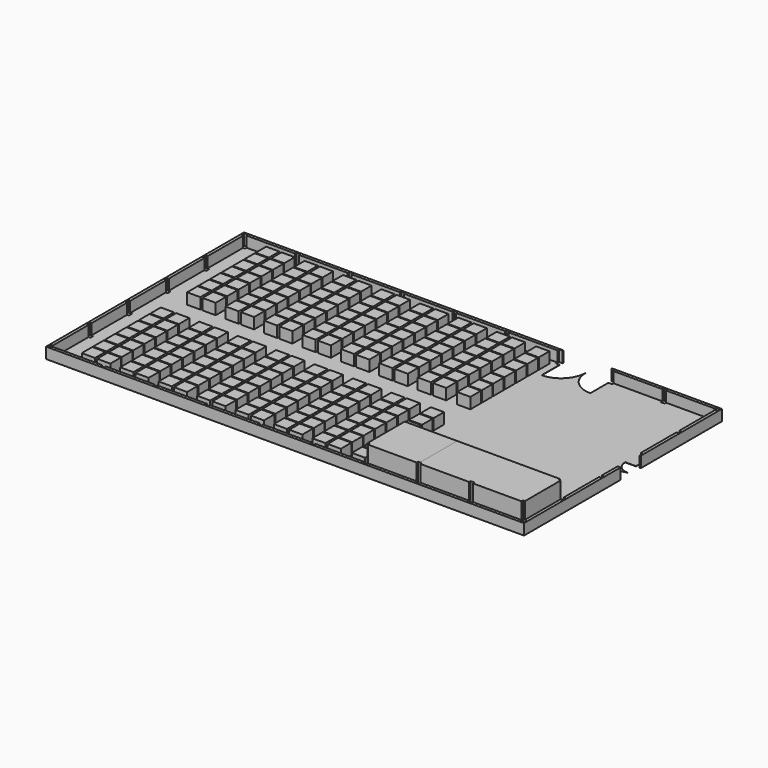
from build123d import *

# Parameters (mm, degrees)
F1_DEPTH = 25
F2_DEPTH = 2500
F3_DEPTH = 2500
F4_DEPTH = 1000
F5_W     = 1200
F5_H     = 1200
F6_DEPTH = 1000


# Not quite as in the source:
# - a feature names something its author has since deleted; it is built from what else it names


with BuildPart() as f1:
    # F0 (on Top) → F1 (new body)
    with BuildSketch(Plane.XY):
        Polygon((28666.6668, 170), (28666.6668, 4400), (28666.6668, 10000), (0, 10000), (0, 8970), (170, 8970), (170, 8630), (0, 8630), (0, 4570), (170, 4570), (170, 4230), (0, 4230), (0, 170), (170, 170), (170, 0), (4607.7778, 0), (4607.7778, 170), (4947.7778, 170), (4947.7778, 0), (9385.5556, 0), (9385.5556, 170), (9725.5556, 170), (9725.5556, 0), (14163.3334, 0), (14163.3334, 170), (14503.3334, 170), (14503.3334, 0), (18941.1112, 0), (18941.1112, 170), (19281.1112, 170), (19281.1112, 0), (23718.889, 0), (23718.889, 170), (24058.889, 170), (24058.889, 0), (28496.6668, 0), (28496.6668, 170), align=None)
        with BuildLine():
            ThreePointArc((33274.4446, 19781.1111), (31705.4532121104, 20431.0086121104), (31055.5557, 22000))
            ThreePointArc((31055.5557, 22000), (30405.6581878896, 20431.0086121104), (28836.6668, 19781.1111))
            Line((28836.6668, 19781.1111), (28836.6668, 21830))
            Line((28836.6668, 21830), (28496.6668, 21830))
            Line((28496.6668, 21830), (28496.6668, 22000))
            Line((28496.6668, 22000), (24058.889, 22000))
            Line((24058.889, 22000), (24058.889, 21830))
            Line((24058.889, 21830), (23718.889, 21830))
            Line((23718.889, 21830), (23718.889, 22000))
            Line((23718.889, 22000), (19281.1112, 22000))
            Line((19281.1112, 22000), (19281.1112, 21830))
            Line((19281.1112, 21830), (18941.1112, 21830))
            Line((18941.1112, 21830), (18941.1112, 22000))
            Line((18941.1112, 22000), (14503.3334, 22000))
            Line((14503.3334, 22000), (14503.3334, 21830))
            Line((14503.3334, 21830), (14163.3334, 21830))
            Line((14163.3334, 21830), (14163.3334, 22000))
            Line((14163.3334, 22000), (9725.5556, 22000))
            Line((9725.5556, 22000), (9725.5556, 21830))
            Line((9725.5556, 21830), (9385.5556, 21830))
            Line((9385.5556, 21830), (9385.5556, 22000))
            Line((9385.5556, 22000), (4947.7778, 22000))
            Line((4947.7778, 22000), (4947.7778, 21830))
            Line((4947.7778, 21830), (4607.7778, 21830))
            Line((4607.7778, 21830), (4607.7778, 22000))
            Line((4607.7778, 22000), (170, 22000))
            Line((170, 22000), (170, 21830))
            Line((170, 21830), (0, 21830))
            Line((0, 21830), (0, 17770))
            Line((0, 17770), (170, 17770))
            Line((170, 17770), (170, 17430))
            Line((170, 17430), (0, 17430))
            Line((0, 17430), (0, 13370))
            Line((0, 13370), (170, 13370))
            Line((170, 13370), (170, 13030))
            Line((170, 13030), (0, 13030))
            Line((0, 13030), (0, 12000))
            Line((0, 12000), (0, 10000))
            Line((0, 10000), (28666.6668, 10000))
            Line((28666.6668, 10000), (28666.6668, 4400))
            Line((28666.6668, 4400), (33444.4446, 4400))
            Line((33444.4446, 4400), (42830, 4400))
            Line((42830, 4400), (42830, 4570))
            Line((42830, 4570), (43000, 4570))
            Line((43000, 4570), (43000, 8630))
            Line((43000, 8630), (42830, 8630))
            Line((42830, 8630), (42830, 8970))
            Line((42830, 8970), (43000, 8970))
            Line((43000, 8970), (43000, 10730))
            Line((43000, 10730), (41850, 10730))
            ThreePointArc((41850, 10730), (42186.8272016355, 11543.1727983645), (43000, 11880))
            ThreePointArc((43000, 11880), (42186.8272016355, 12216.8272016355), (41850, 13030))
            Line((41850, 13030), (42830, 13030))
            Line((42830, 13030), (42830, 13370))
            Line((42830, 13370), (43000, 13370))
            Line((43000, 13370), (43000, 17430))
            Line((43000, 17430), (42830, 17430))
            Line((42830, 17430), (42830, 17770))
            Line((42830, 17770), (43000, 17770))
            Line((43000, 17770), (43000, 21830))
            Line((43000, 21830), (42830.0002, 21830))
            Line((42830.0002, 21830), (42830.0002, 22000))
            Line((42830.0002, 22000), (38392.2224, 22000))
            Line((38392.2224, 22000), (38392.2224, 21830))
            Line((38392.2224, 21830), (38052.2224, 21830))
            Line((38052.2224, 21830), (38052.2224, 22000))
            Line((38052.2224, 22000), (33614.4446, 22000))
            Line((33614.4446, 22000), (33614.4446, 21830))
            Line((33614.4446, 21830), (33274.4446, 21830))
            Line((33274.4446, 21830), (33274.4446, 19781.1111))
        make_face()
    extrude(amount=F1_DEPTH)

    # F0 (on Top) → F4 (join)
    with BuildSketch(Plane.XY):
        Polygon((24058.889, 22000), (28496.6668, 22000), (28496.6668, 22170), (28836.6668, 22170), (28836.6668, 22270), (-270, 22270), (-270, -270), (43270.0002, -270), (43270.0002, 10730), (43000, 10730), (43000, 8970), (43170, 8970), (43170, 8630), (43000, 8630), (43000, 4570), (43170, 4570), (43170, 4230), (43000.0000077273, 4230), (43000.0001922727, 170), (43170.0002, 170), (43170.0002, -170), (42830.0002, -170), (42830.0002, 0), (38392.2224, 0), (38392.2224, -170), (38052.2224, -170), (38052.2224, 0), (33614.4446, 0), (33614.4446, -170), (33274.4446, -170), (33274.4446, 0), (28836.6668, 0), (28836.6668, -170), (28496.6668, -170), (28496.6668, 0), (24058.889, 0), (24058.889, -170), (23718.889, -170), (23718.889, 0), (19281.1112, 0), (19281.1112, -170), (18941.1112, -170), (18941.1112, 0), (14503.3334, 0), (14503.3334, -170), (14163.3334, -170), (14163.3334, 0), (9725.5556, 0), (9725.5556, -170), (9385.5556, -170), (9385.5556, 0), (4947.7778, 0), (4947.7778, -170), (4607.7778, -170), (4607.7778, 0), (170, 0), (170, -170), (-170, -170), (-170, 170), (0, 170), (0, 4230), (-170, 4230), (-170, 4570), (0, 4570), (0, 8630), (-170, 8630), (-170, 8970), (0, 8970), (0, 10000), (0, 12000), (0, 13030), (-170, 13030), (-170, 13370), (0, 13370), (0, 17430), (-170, 17430), (-170, 17770), (0, 17770), (0, 21830), (-170, 21830), (-170, 22170), (170, 22170), (170, 22000), (4607.7778, 22000), (4607.7778, 22170), (4947.7778, 22170), (4947.7778, 22000), (9385.5556, 22000), (9385.5556, 22170), (9725.5556, 22170), (9725.5556, 22000), (14163.3334, 22000), (14163.3334, 22170), (14503.3334, 22170), (14503.3334, 22000), (18941.1112, 22000), (18941.1112, 22170), (19281.1112, 22170), (19281.1112, 22000), (23718.889, 22000), (23718.889, 22170), (24058.889, 22170), align=None)
        Polygon((33614.4446, 22170), (33614.4446, 22000), (38052.2224, 22000), (38052.2224, 22170), (38392.2224, 22170), (38392.2224, 22000), (42830.0002, 22000), (42830.0002, 22170), (43170.0002, 22170), (43170.0002, 21830), (43000, 21830), (43000, 17770), (43170, 17770), (43170, 17430), (43000, 17430), (43000, 13370), (43170, 13370), (43170, 13030), (43270.0002, 13030), (43270.0002, 22270), (33274.4446, 22270), (33274.4446, 22170), align=None)
    extrude(amount=F4_DEPTH)

    # F5 (on face) → F6 (join)
    with BuildSketch(Plane.XY.offset(25)):
        with Locations((27566.6668, 1100)):
            Rectangle(F5_W, F5_H)
        with Locations((27566.6668, 2400)):
            Rectangle(F5_W, F5_H)
        with Locations((27566.6668, 3700)):
            Rectangle(F5_W, F5_H)
        with Locations((27566.6668, 5000)):
            Rectangle(F5_W, F5_H)
        with Locations((27566.6668, 6300)):
            Rectangle(F5_W, F5_H)
        with Locations((27566.6668, 7600)):
            Rectangle(F5_W, F5_H)
        with Locations((27566.6668, 8900)):
            Rectangle(F5_W, F5_H)
        with Locations((25366.6668, 1100)):
            Rectangle(F5_W, F5_H)
        with Locations((23966.6668, 1100)):
            Rectangle(F5_W, F5_H)
        with Locations((21866.6668, 1100)):
            Rectangle(F5_W, F5_H)
        with Locations((20466.6668, 1100)):
            Rectangle(F5_W, F5_H)
        with Locations((18366.6668, 1100)):
            Rectangle(F5_W, F5_H)
        with Locations((16966.6668, 1100)):
            Rectangle(F5_W, F5_H)
        with Locations((14866.6668, 1100)):
            Rectangle(F5_W, F5_H)
        with Locations((13466.6668, 1100)):
            Rectangle(F5_W, F5_H)
        with Locations((11366.6668, 1100)):
            Rectangle(F5_W, F5_H)
        with Locations((9966.6668, 1100)):
            Rectangle(F5_W, F5_H)
        with Locations((7866.6668, 1100)):
            Rectangle(F5_W, F5_H)
        with Locations((6466.6668, 1100)):
            Rectangle(F5_W, F5_H)
        with Locations((4366.6668, 1100)):
            Rectangle(F5_W, F5_H)
        with Locations((2966.6668, 1100)):
            Rectangle(F5_W, F5_H)
        with Locations((18366.6668, 2400)):
            Rectangle(F5_W, F5_H)
        with Locations((23966.6668, 2400)):
            Rectangle(F5_W, F5_H)
        with Locations((14866.6668, 2400)):
            Rectangle(F5_W, F5_H)
        with Locations((2966.6668, 2400)):
            Rectangle(F5_W, F5_H)
        with Locations((13466.6668, 2400)):
            Rectangle(F5_W, F5_H)
        with Locations((9966.6668, 2400)):
            Rectangle(F5_W, F5_H)
        with Locations((11366.6668, 2400)):
            Rectangle(F5_W, F5_H)
        with Locations((25366.6668, 2400)):
            Rectangle(F5_W, F5_H)
        with Locations((6466.6668, 2400)):
            Rectangle(F5_W, F5_H)
        with Locations((16966.6668, 2400)):
            Rectangle(F5_W, F5_H)
        with Locations((7866.6668, 2400)):
            Rectangle(F5_W, F5_H)
        with Locations((20466.6668, 2400)):
            Rectangle(F5_W, F5_H)
        with Locations((21866.6668, 2400)):
            Rectangle(F5_W, F5_H)
        with Locations((4366.6668, 2400)):
            Rectangle(F5_W, F5_H)
        with Locations((18366.6668, 3700)):
            Rectangle(F5_W, F5_H)
        with Locations((23966.6668, 3700)):
            Rectangle(F5_W, F5_H)
        with Locations((14866.6668, 3700)):
            Rectangle(F5_W, F5_H)
        with Locations((2966.6668, 3700)):
            Rectangle(F5_W, F5_H)
        with Locations((13466.6668, 3700)):
            Rectangle(F5_W, F5_H)
        with Locations((9966.6668, 3700)):
            Rectangle(F5_W, F5_H)
        with Locations((11366.6668, 3700)):
            Rectangle(F5_W, F5_H)
        with Locations((25366.6668, 3700)):
            Rectangle(F5_W, F5_H)
        with Locations((6466.6668, 3700)):
            Rectangle(F5_W, F5_H)
        with Locations((16966.6668, 3700)):
            Rectangle(F5_W, F5_H)
        with Locations((7866.6668, 3700)):
            Rectangle(F5_W, F5_H)
        with Locations((20466.6668, 3700)):
            Rectangle(F5_W, F5_H)
        with Locations((21866.6668, 3700)):
            Rectangle(F5_W, F5_H)
        with Locations((4366.6668, 3700)):
            Rectangle(F5_W, F5_H)
        with Locations((18366.6668, 5000)):
            Rectangle(F5_W, F5_H)
        with Locations((23966.6668, 5000)):
            Rectangle(F5_W, F5_H)
        with Locations((14866.6668, 5000)):
            Rectangle(F5_W, F5_H)
        with Locations((2966.6668, 5000)):
            Rectangle(F5_W, F5_H)
        with Locations((13466.6668, 5000)):
            Rectangle(F5_W, F5_H)
        with Locations((9966.6668, 5000)):
            Rectangle(F5_W, F5_H)
        with Locations((11366.6668, 5000)):
            Rectangle(F5_W, F5_H)
        with Locations((25366.6668, 5000)):
            Rectangle(F5_W, F5_H)
        with Locations((6466.6668, 5000)):
            Rectangle(F5_W, F5_H)
        with Locations((16966.6668, 5000)):
            Rectangle(F5_W, F5_H)
        with Locations((7866.6668, 5000)):
            Rectangle(F5_W, F5_H)
        with Locations((20466.6668, 5000)):
            Rectangle(F5_W, F5_H)
        with Locations((21866.6668, 5000)):
            Rectangle(F5_W, F5_H)
        with Locations((4366.6668, 5000)):
            Rectangle(F5_W, F5_H)
        with Locations((18366.6668, 6300)):
            Rectangle(F5_W, F5_H)
        with Locations((23966.6668, 6300)):
            Rectangle(F5_W, F5_H)
        with Locations((14866.6668, 6300)):
            Rectangle(F5_W, F5_H)
        with Locations((2966.6668, 6300)):
            Rectangle(F5_W, F5_H)
        with Locations((13466.6668, 6300)):
            Rectangle(F5_W, F5_H)
        with Locations((9966.6668, 6300)):
            Rectangle(F5_W, F5_H)
        with Locations((11366.6668, 6300)):
            Rectangle(F5_W, F5_H)
        with Locations((25366.6668, 6300)):
            Rectangle(F5_W, F5_H)
        with Locations((6466.6668, 6300)):
            Rectangle(F5_W, F5_H)
        with Locations((16966.6668, 6300)):
            Rectangle(F5_W, F5_H)
        with Locations((7866.6668, 6300)):
            Rectangle(F5_W, F5_H)
        with Locations((20466.6668, 6300)):
            Rectangle(F5_W, F5_H)
        with Locations((21866.6668, 6300)):
            Rectangle(F5_W, F5_H)
        with Locations((4366.6668, 6300)):
            Rectangle(F5_W, F5_H)
        with Locations((18366.6668, 7600)):
            Rectangle(F5_W, F5_H)
        with Locations((23966.6668, 7600)):
            Rectangle(F5_W, F5_H)
        with Locations((14866.6668, 7600)):
            Rectangle(F5_W, F5_H)
        with Locations((2966.6668, 7600)):
            Rectangle(F5_W, F5_H)
        with Locations((13466.6668, 7600)):
            Rectangle(F5_W, F5_H)
        with Locations((9966.6668, 7600)):
            Rectangle(F5_W, F5_H)
        with Locations((11366.6668, 7600)):
            Rectangle(F5_W, F5_H)
        with Locations((25366.6668, 7600)):
            Rectangle(F5_W, F5_H)
        with Locations((6466.6668, 7600)):
            Rectangle(F5_W, F5_H)
        with Locations((16966.6668, 7600)):
            Rectangle(F5_W, F5_H)
        with Locations((7866.6668, 7600)):
            Rectangle(F5_W, F5_H)
        with Locations((20466.6668, 7600)):
            Rectangle(F5_W, F5_H)
        with Locations((21866.6668, 7600)):
            Rectangle(F5_W, F5_H)
        with Locations((4366.6668, 7600)):
            Rectangle(F5_W, F5_H)
        with Locations((18366.6668, 8900)):
            Rectangle(F5_W, F5_H)
        with Locations((23966.6668, 8900)):
            Rectangle(F5_W, F5_H)
        with Locations((14866.6668, 8900)):
            Rectangle(F5_W, F5_H)
        with Locations((2966.6668, 8900)):
            Rectangle(F5_W, F5_H)
        with Locations((13466.6668, 8900)):
            Rectangle(F5_W, F5_H)
        with Locations((9966.6668, 8900)):
            Rectangle(F5_W, F5_H)
        with Locations((11366.6668, 8900)):
            Rectangle(F5_W, F5_H)
        with Locations((25366.6668, 8900)):
            Rectangle(F5_W, F5_H)
        with Locations((6466.6668, 8900)):
            Rectangle(F5_W, F5_H)
        with Locations((16966.6668, 8900)):
            Rectangle(F5_W, F5_H)
        with Locations((7866.6668, 8900)):
            Rectangle(F5_W, F5_H)
        with Locations((20466.6668, 8900)):
            Rectangle(F5_W, F5_H)
        with Locations((21866.6668, 8900)):
            Rectangle(F5_W, F5_H)
        with Locations((4366.6668, 8900)):
            Rectangle(F5_W, F5_H)
        with Locations((20466.6668, 17000)):
            Rectangle(F5_W, F5_H)
        with Locations((21866.6668, 20900)):
            Rectangle(F5_W, F5_H)
        with Locations((21866.6668, 17000)):
            Rectangle(F5_W, F5_H)
        with Locations((20466.6668, 18300)):
            Rectangle(F5_W, F5_H)
        with Locations((21866.6668, 13100)):
            Rectangle(F5_W, F5_H)
        with Locations((2966.6668, 20900)):
            Rectangle(F5_W, F5_H)
        with Locations((20466.6668, 13100)):
            Rectangle(F5_W, F5_H)
        with Locations((21866.6668, 14400)):
            Rectangle(F5_W, F5_H)
        with Locations((27566.6668, 19600)):
            Rectangle(F5_W, F5_H)
        with Locations((21866.6668, 15700)):
            Rectangle(F5_W, F5_H)
        with Locations((23966.6668, 19600)):
            Rectangle(F5_W, F5_H)
        with Locations((20466.6668, 14400)):
            Rectangle(F5_W, F5_H)
        with Locations((21866.6668, 19600)):
            Rectangle(F5_W, F5_H)
        with Locations((20466.6668, 15700)):
            Rectangle(F5_W, F5_H)
        with Locations((20466.6668, 19600)):
            Rectangle(F5_W, F5_H)
        with Locations((27566.6668, 20900)):
            Rectangle(F5_W, F5_H)
        with Locations((20466.6668, 20900)):
            Rectangle(F5_W, F5_H)
        with Locations((21866.6668, 18300)):
            Rectangle(F5_W, F5_H)
        with Locations((11366.6668, 18300)):
            Rectangle(F5_W, F5_H)
        with Locations((25366.6668, 17000)):
            Rectangle(F5_W, F5_H)
        with Locations((6466.6668, 15700)):
            Rectangle(F5_W, F5_H)
        with Locations((2966.6668, 17000)):
            Rectangle(F5_W, F5_H)
        with Locations((6466.6668, 13100)):
            Rectangle(F5_W, F5_H)
        with Locations((11366.6668, 20900)):
            Rectangle(F5_W, F5_H)
        with Locations((11366.6668, 15700)):
            Rectangle(F5_W, F5_H)
        with Locations((25366.6668, 19600)):
            Rectangle(F5_W, F5_H)
        with Locations((14866.6668, 14400)):
            Rectangle(F5_W, F5_H)
        with Locations((27566.6668, 17000)):
            Rectangle(F5_W, F5_H)
        with Locations((16966.6668, 15700)):
            Rectangle(F5_W, F5_H)
        with Locations((18366.6668, 17000)):
            Rectangle(F5_W, F5_H)
        with Locations((18366.6668, 19600)):
            Rectangle(F5_W, F5_H)
        with Locations((16966.6668, 18300)):
            Rectangle(F5_W, F5_H)
        with Locations((6466.6668, 17000)):
            Rectangle(F5_W, F5_H)
        with Locations((2966.6668, 13100)):
            Rectangle(F5_W, F5_H)
        with Locations((2966.6668, 18300)):
            Rectangle(F5_W, F5_H)
        with Locations((18366.6668, 13100)):
            Rectangle(F5_W, F5_H)
        with Locations((16966.6668, 14400)):
            Rectangle(F5_W, F5_H)
        with Locations((7866.6668, 19600)):
            Rectangle(F5_W, F5_H)
        with Locations((6466.6668, 20900)):
            Rectangle(F5_W, F5_H)
        with Locations((13466.6668, 17000)):
            Rectangle(F5_W, F5_H)
        with Locations((23966.6668, 14400)):
            Rectangle(F5_W, F5_H)
        with Locations((2966.6668, 14400)):
            Rectangle(F5_W, F5_H)
        with Locations((18366.6668, 14400)):
            Rectangle(F5_W, F5_H)
        with Locations((9966.6668, 17000)):
            Rectangle(F5_W, F5_H)
        with Locations((4366.6668, 15700)):
            Rectangle(F5_W, F5_H)
        with Locations((23966.6668, 17000)):
            Rectangle(F5_W, F5_H)
        with Locations((9966.6668, 15700)):
            Rectangle(F5_W, F5_H)
        with Locations((27566.6668, 18300)):
            Rectangle(F5_W, F5_H)
        with Locations((7866.6668, 17000)):
            Rectangle(F5_W, F5_H)
        with Locations((18366.6668, 15700)):
            Rectangle(F5_W, F5_H)
        with Locations((14866.6668, 15700)):
            Rectangle(F5_W, F5_H)
        with Locations((27566.6668, 14400)):
            Rectangle(F5_W, F5_H)
        with Locations((13466.6668, 15700)):
            Rectangle(F5_W, F5_H)
        with Locations((7866.6668, 15700)):
            Rectangle(F5_W, F5_H)
        with Locations((14866.6668, 18300)):
            Rectangle(F5_W, F5_H)
        with Locations((13466.6668, 13100)):
            Rectangle(F5_W, F5_H)
        with Locations((14866.6668, 20900)):
            Rectangle(F5_W, F5_H)
        with Locations((2966.6668, 15700)):
            Rectangle(F5_W, F5_H)
        with Locations((7866.6668, 18300)):
            Rectangle(F5_W, F5_H)
        with Locations((27566.6668, 13100)):
            Rectangle(F5_W, F5_H)
        with Locations((25366.6668, 20900)):
            Rectangle(F5_W, F5_H)
        with Locations((9966.6668, 13100)):
            Rectangle(F5_W, F5_H)
        with Locations((4366.6668, 19600)):
            Rectangle(F5_W, F5_H)
        with Locations((11366.6668, 13100)):
            Rectangle(F5_W, F5_H)
        with Locations((6466.6668, 14400)):
            Rectangle(F5_W, F5_H)
        with Locations((6466.6668, 19600)):
            Rectangle(F5_W, F5_H)
        with Locations((13466.6668, 19600)):
            Rectangle(F5_W, F5_H)
        with Locations((25366.6668, 15700)):
            Rectangle(F5_W, F5_H)
        with Locations((14866.6668, 13100)):
            Rectangle(F5_W, F5_H)
        with Locations((13466.6668, 20900)):
            Rectangle(F5_W, F5_H)
        with Locations((23966.6668, 15700)):
            Rectangle(F5_W, F5_H)
        with Locations((23966.6668, 13100)):
            Rectangle(F5_W, F5_H)
        with Locations((11366.6668, 17000)):
            Rectangle(F5_W, F5_H)
        with Locations((11366.6668, 19600)):
            Rectangle(F5_W, F5_H)
        with Locations((9966.6668, 19600)):
            Rectangle(F5_W, F5_H)
        with Locations((27566.6668, 15700)):
            Rectangle(F5_W, F5_H)
        with Locations((4366.6668, 14400)):
            Rectangle(F5_W, F5_H)
        with Locations((13466.6668, 18300)):
            Rectangle(F5_W, F5_H)
        with Locations((18366.6668, 20900)):
            Rectangle(F5_W, F5_H)
        with Locations((14866.6668, 17000)):
            Rectangle(F5_W, F5_H)
        with Locations((4366.6668, 20900)):
            Rectangle(F5_W, F5_H)
        with Locations((6466.6668, 18300)):
            Rectangle(F5_W, F5_H)
        with Locations((7866.6668, 14400)):
            Rectangle(F5_W, F5_H)
        with Locations((13466.6668, 14400)):
            Rectangle(F5_W, F5_H)
        with Locations((11366.6668, 14400)):
            Rectangle(F5_W, F5_H)
        with Locations((9966.6668, 18300)):
            Rectangle(F5_W, F5_H)
        with Locations((16966.6668, 13100)):
            Rectangle(F5_W, F5_H)
        with Locations((16966.6668, 20900)):
            Rectangle(F5_W, F5_H)
        with Locations((23966.6668, 20900)):
            Rectangle(F5_W, F5_H)
        with Locations((16966.6668, 19600)):
            Rectangle(F5_W, F5_H)
        with Locations((9966.6668, 14400)):
            Rectangle(F5_W, F5_H)
        with Locations((25366.6668, 18300)):
            Rectangle(F5_W, F5_H)
        with Locations((25366.6668, 14400)):
            Rectangle(F5_W, F5_H)
        with Locations((25366.6668, 13100)):
            Rectangle(F5_W, F5_H)
        with Locations((7866.6668, 13100)):
            Rectangle(F5_W, F5_H)
        with Locations((18366.6668, 18300)):
            Rectangle(F5_W, F5_H)
        with Locations((16966.6668, 17000)):
            Rectangle(F5_W, F5_H)
        with Locations((7866.6668, 20900)):
            Rectangle(F5_W, F5_H)
        with Locations((2966.6668, 19600)):
            Rectangle(F5_W, F5_H)
        with Locations((23966.6668, 18300)):
            Rectangle(F5_W, F5_H)
        with Locations((4366.6668, 17000)):
            Rectangle(F5_W, F5_H)
        with Locations((9966.6668, 20900)):
            Rectangle(F5_W, F5_H)
        with Locations((4366.6668, 13100)):
            Rectangle(F5_W, F5_H)
        with Locations((4366.6668, 18300)):
            Rectangle(F5_W, F5_H)
        with Locations((14866.6668, 19600)):
            Rectangle(F5_W, F5_H)
    extrude(amount=F6_DEPTH)


with BuildPart() as f2:
    # F0 (on Top) → F2 (new body)
    with BuildSketch(Plane.XY):
        Polygon((43000.0001922727, 170), (43000.0000077273, 4230), (42830, 4230), (42830, 4400), (33444.4446, 4400), (33444.4446, 170), (33614.4446, 170), (33614.4446, 0), (38052.2224, 0), (38052.2224, 170), (38392.2224, 170), (38392.2224, 0), (42830.0002, 0), (42830.0002, 170), align=None)
    extrude(amount=F2_DEPTH)


with BuildPart() as f3:
    # F0 (on Top) → F3 (new body)
    with BuildSketch(Plane.XY):
        Polygon((33444.4446, 170), (33444.4446, 4400), (28666.6668, 4400), (28666.6668, 170), (28836.6668, 170), (28836.6668, 0), (33274.4446, 0), (33274.4446, 170), align=None)
    extrude(amount=F3_DEPTH)


solid = Compound([f1.part, f2.part, f3.part])
